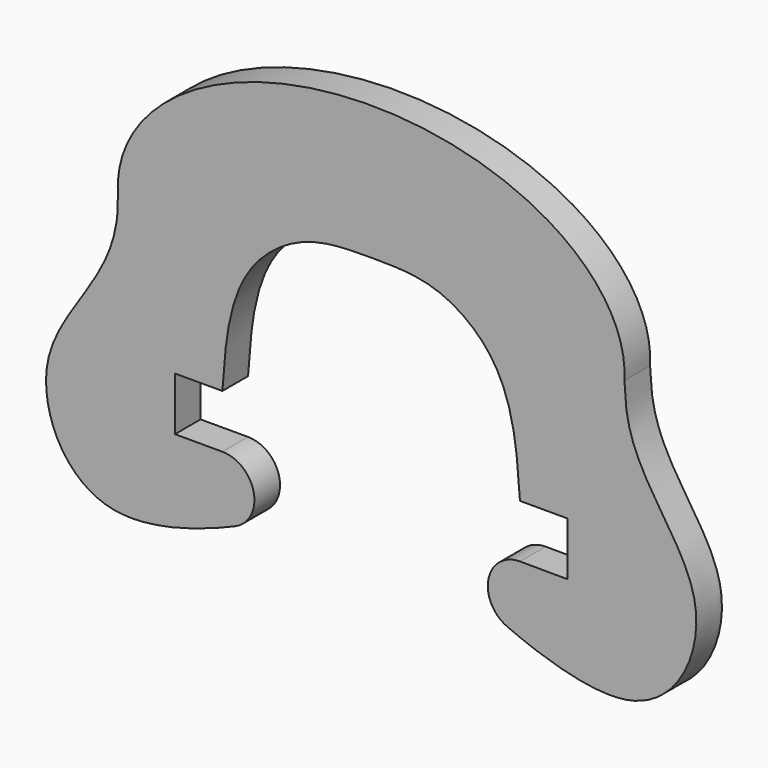
from build123d import *

# Parameters (mm, degrees)
F1_DEPTH = 3


# Not quite as in the source:
# - ends of sketch curves that miss each other by under 0.0002 mm in the source are joined
# - the dataset's text gives a spline's control points without its knots; the knots are read off the source's solid


with BuildPart() as f1:
    # F0 (on Front) → F1 (new body)
    with BuildSketch(Plane.XZ):
        with BuildLine():
            Line((-13.923003, -12.408035), (-18.356865, -12.408035))
            Line((-18.356865, -12.408035), (-18.356865, -7.408035))
            Line((-18.356865, -7.408035), (-13.918449, -7.407196))
            add(Edge.make_bspline(
                [(-13.918449, -7.407196), (-13.638513, -3.334265), (-13.208401, 2.923662), (-6.220814, 8.085581), (-2.060784, 8.094994), (-0.001865, 8.099652)],
                knots=[0, 0, 0, 0, 11.557339, 17.757478, 23.833112, 23.833112, 23.833112, 23.833112], degree=3))
            add(Edge.make_bspline(
                [(13.914719, -7.407196), (13.634783, -3.334265), (13.20467, 2.923662), (6.217083, 8.085581), (2.057053, 8.094994), (-0.001865, 8.099652)],
                knots=[0, 0, 0, 0, 11.557339, 17.757478, 23.833112, 23.833112, 23.833112, 23.833112], degree=3))
            Line((13.914719, -7.407196), (18.353135, -7.408035))
            Line((18.353135, -7.408035), (18.353135, -12.408035))
            Line((18.353135, -12.408035), (13.919311, -12.389395))
            ThreePointArc((13.919311, -12.389395), (10.9712332753, -14.7704659552), (12.7070690482, -18.1390758896))
            add(Edge.make_bspline(
                [(23.687616, 5.678493), (23.745513, 5.327843), (23.739909, -1.770351), (33.780162, -8.494813), (26.825149, -23.514858), (15.452431, -19.33681), (12.7070690482, -18.1390758896)],
                knots=[26.688985, 26.688985, 26.688985, 26.688985, 28.557776, 42.872008, 54.1154, 62.665306, 62.665306, 62.665306, 62.665306], degree=3))
            add(Edge.make_bspline(
                [(23.687616, 5.678493), (24.5393769355, 20.6396499944), (-0.0018618243, 20.639652), (-24.5431005841, 20.6396540056), (-23.6913461529, 5.6784965777)],
                knots=[6.248471, 6.248471, 6.248471, 7.8539815, 7.8539815, 9.459492, 9.459492, 9.459492], degree=2, weights=[1, 0.694727572, 1, 0.694727572, 1]))
            add(Edge.make_bspline(
                [(-23.6913461529, 5.6784965777), (-23.674634, 5.350356), (-23.698871, -1.747799), (-33.767305, -8.429992), (-26.875499, -23.479143), (-15.485316, -19.348943), (-12.734943, -18.162761)],
                knots=[26.688985, 26.688985, 26.688985, 26.688985, 28.557776, 42.872008, 54.1154, 62.665306, 62.665306, 62.665306, 62.665306], degree=3))
            ThreePointArc((-12.734943, -18.162761), (-10.9849613794, -14.8014779657), (-13.923003, -12.408035))
        make_face()
    extrude(amount=F1_DEPTH)


solid = f1.part
